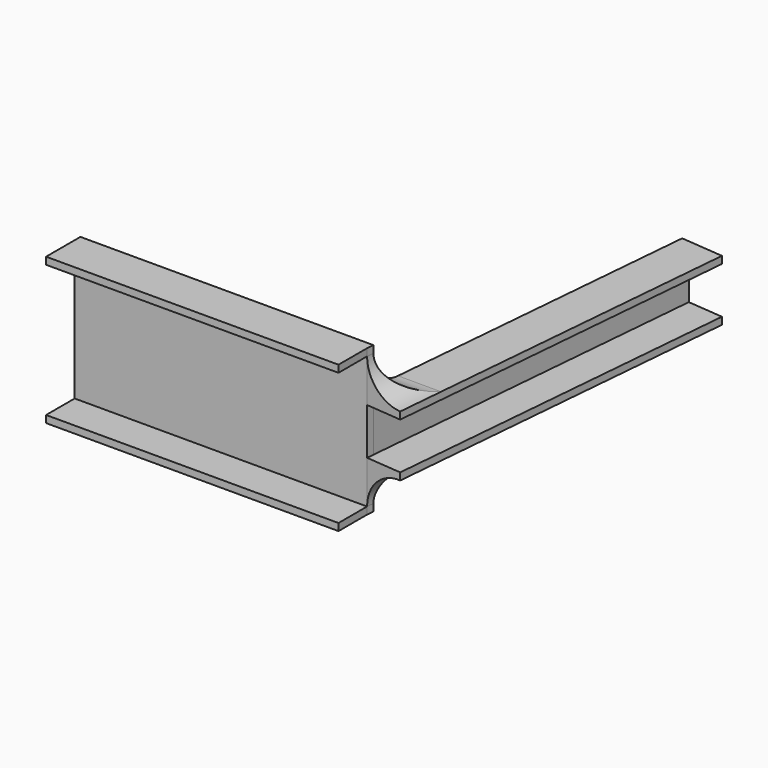
from build123d import *

# Parameters (mm, degrees)
F1_DEPTH = 10.25
F2_DEPTH = 4.25
F4_DEPTH = 5
F5_W     = 40.916331174
F5_H     = 1
F6_DEPTH = 5
F7_R     = 4.99999


# Not quite as in the source:
# - a fillet or chamfer is up to 0.001 mm smaller than in the source, because OpenCascade refuses the exact size


with BuildPart() as f1:
    # F0 (on Top) → F1 (new body, symmetric)
    with BuildSketch(Plane.XY):
        Polygon((0, 0), (-40, 0), (-40, -1), (0.916331174, -1), (1.0038198375, 0), align=None)
    extrude(amount=F1_DEPTH, both=True)

    # F0 (on Top) → F2 (join, symmetric)
    with BuildSketch(Plane.XY):
        Polygon((4.3577871374, 49.8097349046), (0, 0), (1.0038198375, 0), (5.3539818355, 49.7225791618), align=None)
    extrude(amount=F2_DEPTH, both=True)

    # F3 (on face) → F4 (join)
    with BuildSketch(Plane(origin=(0.9961946981, -0.0871557427, 0), x_dir=(0.0871557427, 0.9961946981, 0), z_dir=(0.9961946981, -0.0871557427, 0))):
        Polygon((50, -4.25), (50, -3.25), (-0.916331174, -3.25), (-0.916331174, -4.25), (0.0874886635, -4.25), align=None)
        Polygon((-0.916331174, 3.25), (50, 3.25), (50, 4.25), (0.0874886635, 4.25), (-0.916331174, 4.25), align=None)
    extrude(amount=F4_DEPTH)

    # F5 (on face) → F6 (join)
    with BuildSketch(Plane.XZ.offset(1)):
        with Locations((-19.541834413, 9.75)):
            Rectangle(F5_W, F5_H)
        with Locations((-19.541834413, -9.75)):
            Rectangle(F5_W, F5_H)
    extrude(amount=F6_DEPTH)

    # F7 (radius 5 in the source; OpenCascade refuses exactly that, so slightly less here)
    f7_edges = [f1.edges().sort_by_distance(p)[0] for p in [
        (0.960076, -0.5, -4.25),
        (0.960076, -0.5, 4.25),
        (0.50191, 0, 4.25),
        (0.50191, 0, -4.25),
        (0, 0, 0),
    ]]
    fillet(f7_edges, radius=F7_R)


solid = f1.part
